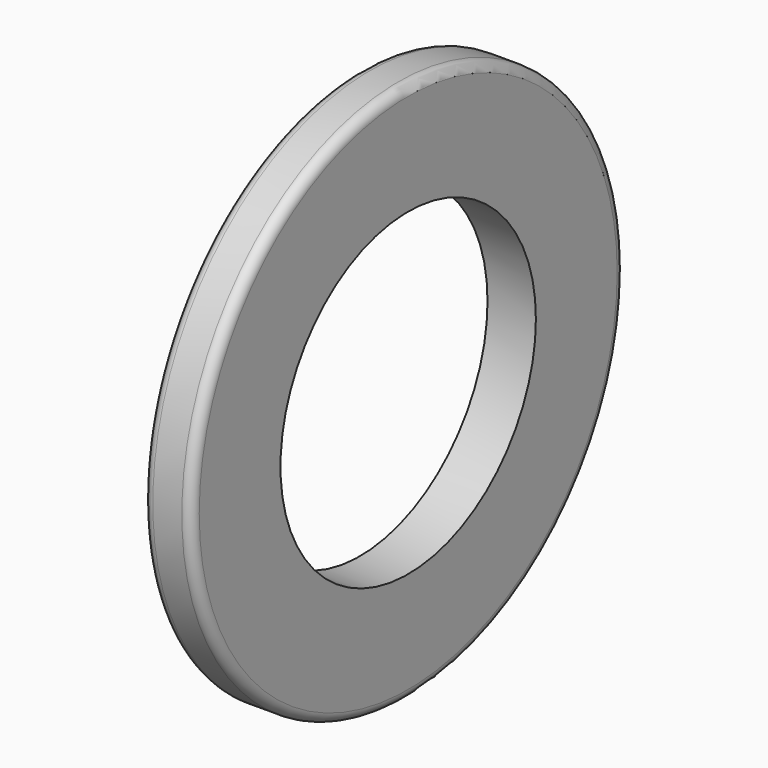
from build123d import *

# Parameters (mm, degrees)
F0_R     = 7
F0_R_2   = 4.125
F1_DEPTH = 1.25
F3_R     = 0.25


# Not quite as in the source:
# - the program builds the solid bodies; features that only make, move or delete a surface that nothing else refers to are left out


with BuildPart() as f1:
    # F0 (on Right) → F1 (new body)
    with BuildSketch(Plane.YZ):
        Circle(F0_R)
        Circle(F0_R_2, mode=Mode.SUBTRACT)
    extrude(amount=F1_DEPTH)

    # F3
    f3_edges = [f1.edges().sort_by_distance(p)[0] for p in [
        (1.25, -7, 0),
        (0, -7, 0),
    ]]
    fillet(f3_edges, radius=F3_R)


solid = f1.part
